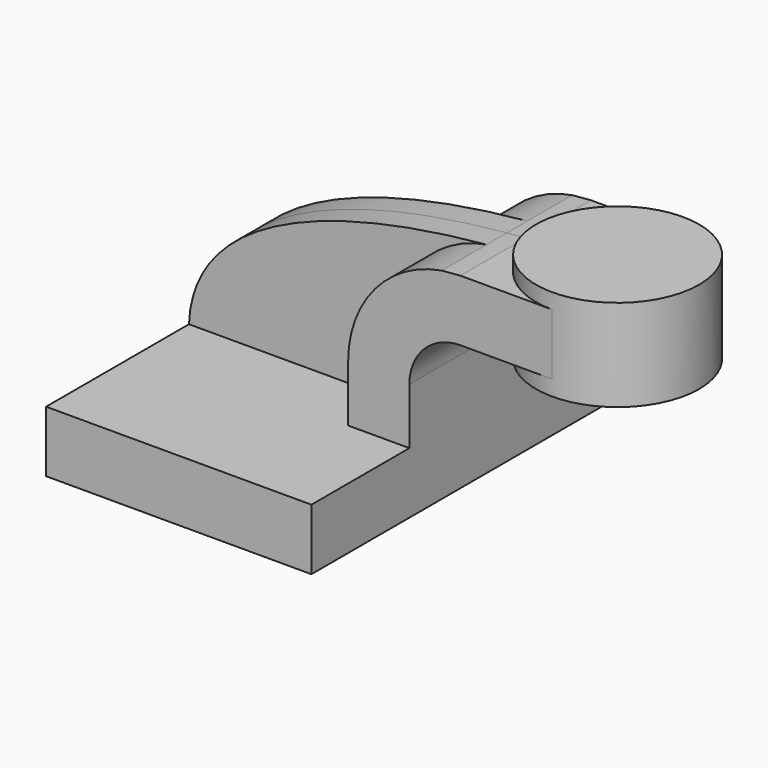
from build123d import *

# Parameters (mm, degrees)
F1_DEPTH = 63.5
F0_W     = 25.4
F0_H     = 19.05
F2_DEPTH = 25.4
F3_DEPTH = 7.9375


with BuildPart() as f1:
    # F0 (on Front) → F1 (new body, symmetric)
    with BuildSketch(Plane.XZ):
        Polygon((41.275, -9.525), (41.275, 9.525), (22.225, 9.525), (-41.275, 9.525), (-41.275, -9.525), align=None)
    extrude(amount=F1_DEPTH, both=True)

    # F0 (on Front) → F2 (join, symmetric)
    with BuildSketch(Plane.XZ):
        with BuildLine():
            Line((22.225, 9.525), (41.275, 9.525))
            Line((41.275, 9.525), (41.275, 27.0002))
            ThreePointArc((41.275, 27.0002), (45.9246798487, 38.2255201513), (57.15, 42.8752))
            Line((57.15, 42.8752), (60.325, 42.8752))
            Line((60.325, 42.8752), (60.325, 61.9252))
            Line((60.325, 61.9252), (57.15, 61.9252))
            add(Edge.make_bspline(
                [(57.15, 61.9252), (55.208694365, 61.7794329693), (53.2677947949, 61.6168749598), (51.3302722534, 61.4369012641)],
                knots=[0, 0, 0, 0, 4.4505519897, 4.4505519897, 4.4505519897, 4.4505519897], degree=3))
            ThreePointArc((51.3302722534, 61.4369012641), (30.4759525329, 49.5446187489), (22.225, 27.0002))
            Line((22.225, 27.0002), (22.225, 9.525))
        make_face()
        with Locations((73.025, 52.4002)):
            Rectangle(F0_W, F0_H)
    extrude(amount=F2_DEPTH, both=True)

    # F0 (on Front) → F3 (join, symmetric)
    with BuildSketch(Plane.XZ):
        with BuildLine():
            Line((-41.275, 9.525), (22.225, 9.525))
            Line((22.225, 9.525), (22.225, 27.0002))
            ThreePointArc((22.225, 27.0002), (30.4759525329, 49.5446187489), (51.3302722534, 61.4369012641))
            add(Edge.make_bspline(
                [(51.3302722534, 61.4369012641), (4.7249280234, 57.1077975465), (-39.9264698354, 42.7019898169), (-41.275, 9.525)],
                knots=[4.4505519897, 4.4505519897, 4.4505519897, 4.4505519897, 111.5045361635, 111.5045361635, 111.5045361635, 111.5045361635], degree=3))
        make_face()
    extrude(amount=F3_DEPTH, both=True)

    # F0 (on Front) → F4 (revolve)
    with BuildSketch(Plane.XZ):
        Polygon((85.725, 61.9252), (85.725, 42.8752), (85.725, 38.1), (111.125, 38.1), (111.125, 66.675), (85.725, 66.675), align=None)
    revolve(axis=Axis((85.725, 0, 52.3875), (0, 0, 1)))


solid = f1.part
